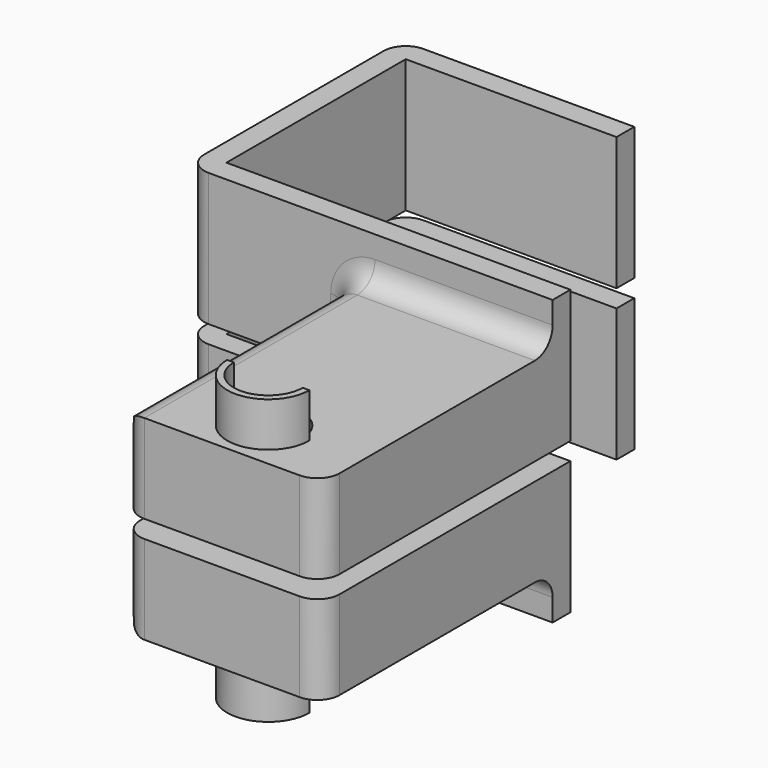
from build123d import *

# Parameters (mm, degrees)
F1_DEPTH  = 30
F2_DEPTH  = 30
F3_W      = 45
F3_H      = 20
F4_DEPTH  = 65
F5_R      = 5
F9_DEPTH  = 10
F10_DEPTH = 10


with BuildPart() as f1:
    # F0 (on Top) → F1 (new body)
    with BuildSketch(Plane.XY):
        Polygon((24.5526876748, 37.0452034771), (-27.9473123252, 37.0452034771), (-27.9473123252, -23.4547965229), (24.5526876748, -23.4547965229), (24.5526876748, -18.4547965229), (19.5526876748, -18.4547965229), (-22.9473123252, -18.4547965229), (-22.9473123252, 32.0452034771), (19.5526876748, 32.0452034771), (24.5526876748, 32.0452034771), align=None)
    extrude(amount=F1_DEPTH)

    # F2 (add): a face of the model
    f2_faces = [f1.faces().sort_by_distance(p)[0] for p in [
        (24.5526876748, -20.9547965229, 15),
    ]]
    extrude(f2_faces, amount=F2_DEPTH)

    # F3 (on face) → F4 (join)
    with BuildSketch(Plane.XZ.offset(23.4547965229)):
        with Locations((32.0526876748, 10)):
            Rectangle(F3_W, F3_H)
    extrude(amount=F4_DEPTH)

    # F5
    f5_edges = [f1.edges().sort_by_distance(p)[0] for p in [
        (-27.947312, -23.454797, 15),
        (9.552688, -55.954797, 20),
        (9.552688, -88.454797, 10),
        (54.552688, -88.454797, 10),
        (-27.947312, 37.045203, 15),
        (9.552688, -23.454797, 10),
        (32.052688, -23.454797, 20),
    ]]
    fillet(f5_edges, radius=F5_R)


with BuildPart() as f7_1:
    # F7: instance of F1
    add(f1.part.mirror(Plane.XY.offset(-2)))


with BuildPart() as f1_1:
    add(f1.part)

    # F8 (on face) → F9 (cut)
    with BuildSketch(Plane.XY.offset(20)):
        with BuildLine():
            Line((33.365637064, -77.0561248064), (41.115637064, -77.0561248064))
            ThreePointArc((41.115637064, -77.0561248064), (33.365637064, -69.3061248064), (25.615637064, -77.0561248064))
            Line((25.615637064, -77.0561248064), (33.365637064, -77.0561248064))
        make_face()
        with BuildLine():
            ThreePointArc((25.615637064, -77.0561248064), (33.365637064, -84.8061248064), (41.115637064, -77.0561248064))
            Line((41.115637064, -77.0561248064), (33.365637064, -77.0561248064))
            Line((33.365637064, -77.0561248064), (25.615637064, -77.0561248064))
        make_face()
    extrude(amount=-F9_DEPTH, mode=Mode.SUBTRACT)

    # F8 (on face) → F10 (join)
    with BuildSketch(Plane.XY.offset(20)):
        with BuildLine():
            Line((42.615637064, -77.0561248064), (41.115637064, -77.0561248064))
            ThreePointArc((41.115637064, -77.0561248064), (33.365637064, -84.8061248064), (25.615637064, -77.0561248064))
            Line((25.615637064, -77.0561248064), (24.115637064, -77.0561248064))
            ThreePointArc((24.115637064, -77.0561248064), (33.365637064, -86.3061248064), (42.615637064, -77.0561248064))
        make_face()
    extrude(amount=F10_DEPTH)


with BuildPart() as f12_1:
    # F12: instance of F1
    add(f1_1.part.mirror(Plane.XY.offset(-2)))


solid = Compound([f1_1.part, f12_1.part])
